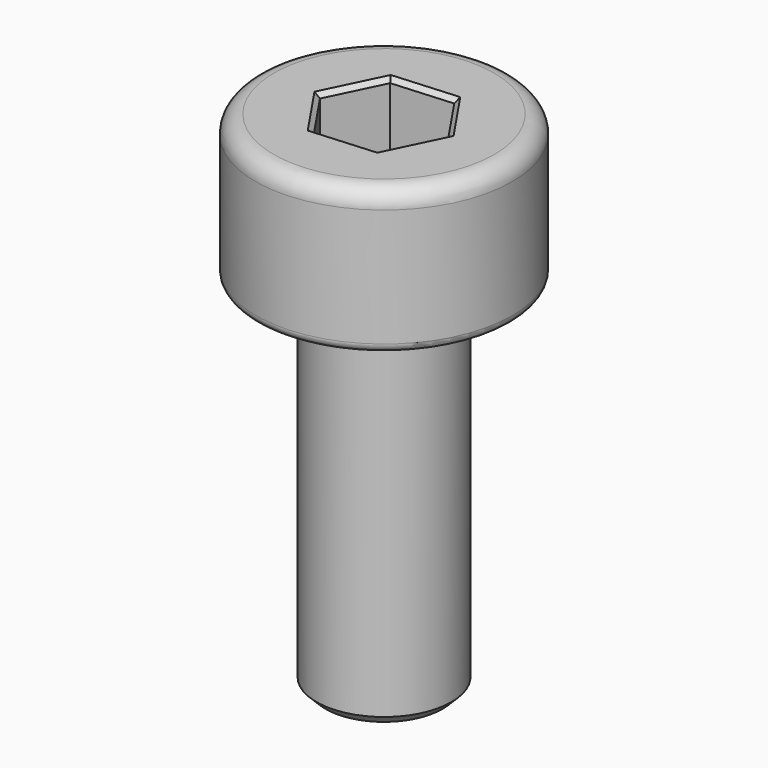
from build123d import *

# Parameters (mm, degrees)
F0_R     = 2.85
F0_R_2   = 1.5
F1_DEPTH = 3.22
F2_DEPTH = 8
F3_R     = 0.4
F4_R     = 0.2
F5_SIZE  = 0.2
F6_START = 1.32
F6_DEPTH = 23.68
F7_SIZE  = 0.1


# Not quite as in the source:
# - an extrude whose draft closes it to a point is written as a loft to that point


with BuildPart() as f1:
    # F0 (on Top) → F1 (new body)
    with BuildSketch(Plane.XY):
        Circle(F0_R)
        Circle(F0_R_2, mode=Mode.SUBTRACT)
        Circle(F0_R_2)
        Polygon((-1.3465408328, -0.0965804618), (-0.7569115498, 1.1178483376), (0.589629283, 1.2144287993), (1.3465408328, 0.0965804618), (0.7569115498, -1.1178483376), (-0.589629283, -1.2144287993), align=None, mode=Mode.SUBTRACT)
        Polygon((0.589629283, 1.2144287993), (-0.7569115498, 1.1178483376), (-1.3465408328, -0.0965804618), (-0.589629283, -1.2144287993), (0.7569115498, -1.1178483376), (1.3465408328, 0.0965804618), align=None)
    extrude(amount=F1_DEPTH)

    # F0 (on Top) → F2 (join)
    with BuildSketch(Plane.XY):
        Circle(F0_R_2)
        Polygon((-1.3465408328, -0.0965804618), (-0.7569115498, 1.1178483376), (0.589629283, 1.2144287993), (1.3465408328, 0.0965804618), (0.7569115498, -1.1178483376), (-0.589629283, -1.2144287993), align=None, mode=Mode.SUBTRACT)
        Polygon((0.589629283, 1.2144287993), (-0.7569115498, 1.1178483376), (-1.3465408328, -0.0965804618), (-0.589629283, -1.2144287993), (0.7569115498, -1.1178483376), (1.3465408328, 0.0965804618), align=None)
    extrude(amount=-F2_DEPTH)

    # F3
    f3_edges = [f1.edges().sort_by_distance(p)[0] for p in [
        (-2.85, 0, 3.22),
    ]]
    fillet(f3_edges, radius=F3_R)

    # F4
    f4_edges = [f1.edges().sort_by_distance(p)[0] for p in [
        (-2.85, 0, 0),
    ]]
    fillet(f4_edges, radius=F4_R)

    # F5
    f5_edges = [f1.edges().sort_by_distance(p)[0] for p in [
        (-1.5, 0, -8),
    ]]
    chamfer(f5_edges, length=F5_SIZE)

    # F0 (on Top) → F6 (cut)
    with BuildSketch(Plane.XY.offset(F6_START)):
        Polygon((0.589629283, 1.2144287993), (-0.7569115498, 1.1178483376), (-1.3465408328, -0.0965804618), (-0.589629283, -1.2144287993), (0.7569115498, -1.1178483376), (1.3465408328, 0.0965804618), align=None)
    extrude(amount=F6_DEPTH, mode=Mode.SUBTRACT)

    # F7
    f7_edges = [f1.edges().sort_by_distance(p)[0] for p in [
        (-1.051726, 0.510634, 3.22),
        (-0.083641, 1.166139, 3.22),
        (0.968085, 0.655505, 3.22),
        (1.051726, -0.510634, 3.22),
        (0.083641, -1.166139, 3.22),
        (-0.968085, -0.655505, 3.22),
    ]]
    chamfer(f7_edges, length=F7_SIZE)

    # F6_face (on face) → F8 section 0
    with BuildSketch(Plane.XY.offset(1.32), mode=Mode.PRIVATE) as f8_s0:
        Polygon((1.3465408328, 0.0965804618), (0.589629283, 1.2144287993), (-0.7569115498, 1.1178483376), (-1.3465408328, -0.0965804618), (-0.589629283, -1.2144287993), (0.7569115498, -1.1178483376), align=None)
    loft([f8_s0.sketch, Vertex(0, 0, 1.217714003)], ruled=True, mode=Mode.SUBTRACT)


solid = f1.part
